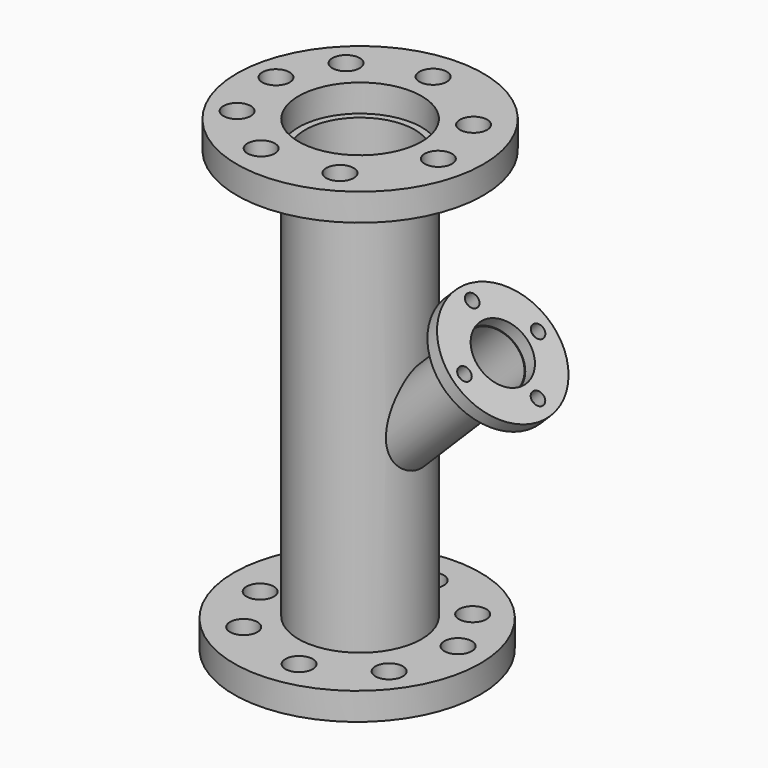
from build123d import *

# Parameters (mm, degrees)
F0_R      = 22.5
F0_R_2    = 20
F1_DEPTH  = 160
F3_R      = 45
F3_R_2    = 22.5
F4_DEPTH  = 10
F2_R      = 45
F2_R_2    = 22.5
F5_DEPTH  = 10
F8_R      = 12
F8_R_2    = 10.7507474001
F9_DEPTH  = 50
F10_R     = 22.5
F10_R_2   = 11
F11_DEPTH = 5
F12_R     = 5
F13_DEPTH = 10
F14_R     = 2.5
F15_DEPTH = 5
F16_R     = 5
F17_DEPTH = 10


# Not quite as in the source:
# - a feature names something its author has since deleted; it is built from what else it names


with BuildPart() as f1:
    # F0 (on Top) → F1 (new body)
    with BuildSketch(Plane.XY):
        Circle(F0_R)
        Circle(F0_R_2, mode=Mode.SUBTRACT)
    extrude(amount=F1_DEPTH)

    # F2 (on Top) → F5 (join)
    with BuildSketch(Plane.XY):
        with Locations((0, -1.3435994042)):
            Circle(F2_R)
        Circle(F2_R_2, mode=Mode.SUBTRACT)
    extrude(amount=F5_DEPTH)

    # F8 (on face) → F9 (join)
    with BuildSketch(Plane(origin=(43.0056799411, 0, 43.0056799411), x_dir=(0, -1, 0), z_dir=(-0.7071067812, 0, -0.7071067812))):
        with Locations((0, 42.075629902)):
            Circle(F8_R)
        with Locations((0, 42.075629902)):
            Circle(F8_R_2, mode=Mode.SUBTRACT)
    extrude(amount=-F9_DEPTH)

    # F10 (on face) → F11 (join)
    with BuildSketch(Plane(origin=(78.3610190004, 0, 78.3610190004), x_dir=(0, 1, 0), z_dir=(0.7071067812, 0, 0.7071067812))):
        with Locations((0, 42.075629902)):
            Circle(F10_R)
        with Locations((0, 42.075629902)):
            Circle(F10_R_2, mode=Mode.SUBTRACT)
    extrude(amount=F11_DEPTH)

    # F14 (on face) → F15 (cut)
    with BuildSketch(Plane(origin=(81.8965529064, 0, 81.8965529064), x_dir=(0, 1, 0), z_dir=(0.7071067812, 0, 0.7071067812))):
        with Locations((16.3939017802, 42.3914864659)):
            Circle(F14_R)
        with Locations((-17.2482132912, 42.37434268)):
            Circle(F14_R)
        with Locations((1.3987645507, 59.4674050808)):
            Circle(F14_R)
        with Locations((1.6441198532, 25.7719922811)):
            Circle(F14_R)
    extrude(amount=-F15_DEPTH, mode=Mode.SUBTRACT)

    # F16 (on face) → F17 (cut)
    with BuildSketch(Plane(origin=(0, 0, 0), x_dir=(1, 0, 0), z_dir=(0, 0, -1))):
        with Locations((1.7036608187, -29.8628024757)):
            Circle(F16_R)
        with Locations((24.2591258138, -21.0912339389)):
            Circle(F16_R)
        with Locations((33.343963325, -3.0781920068)):
            Circle(F16_R)
        with Locations((27.705097571, 21.3568918407)):
            Circle(F16_R)
        with Locations((4.8363660462, 33.8877029717)):
            Circle(F16_R)
        with Locations((-21.7916127294, 25.8993115276)):
            Circle(F16_R)
        with Locations((-31.8162590265, 5.8500124142)):
            Circle(F16_R)
        with Locations((-25.8641205728, -17.3319913447)):
            Circle(F16_R)
    extrude(amount=-F17_DEPTH, mode=Mode.SUBTRACT)


with BuildPart() as f4:
    # F3 (on face) → F4 (new body)
    with BuildSketch(Plane.XY.offset(160)):
        Circle(F3_R)
        Circle(F3_R_2, mode=Mode.SUBTRACT)
    extrude(amount=F4_DEPTH)

    # F12 (on face) → F13 (cut)
    with BuildSketch(Plane.XY.offset(170)):
        with Locations((-30.4371174425, -18.117332831)):
            Circle(F12_R)
        with Locations((-34.7852781415, 5.0728525966)):
            Circle(F12_R)
        with Locations((-10.6288352981, -31.8865031004)):
            Circle(F12_R)
        with Locations((16.4263807237, -29.7124255449)):
            Circle(F12_R)
        with Locations((32.8527614474, -5.3144171834)):
            Circle(F12_R)
        with Locations((27.5383461267, 17.3926390707)):
            Circle(F12_R)
        with Locations((0, 33.3358906209)):
            Circle(F12_R)
        with Locations((-24.6395710856, 24.3980064988)):
            Circle(F12_R)
    extrude(amount=-F13_DEPTH, mode=Mode.SUBTRACT)


solid = Compound([f1.part, f4.part])
